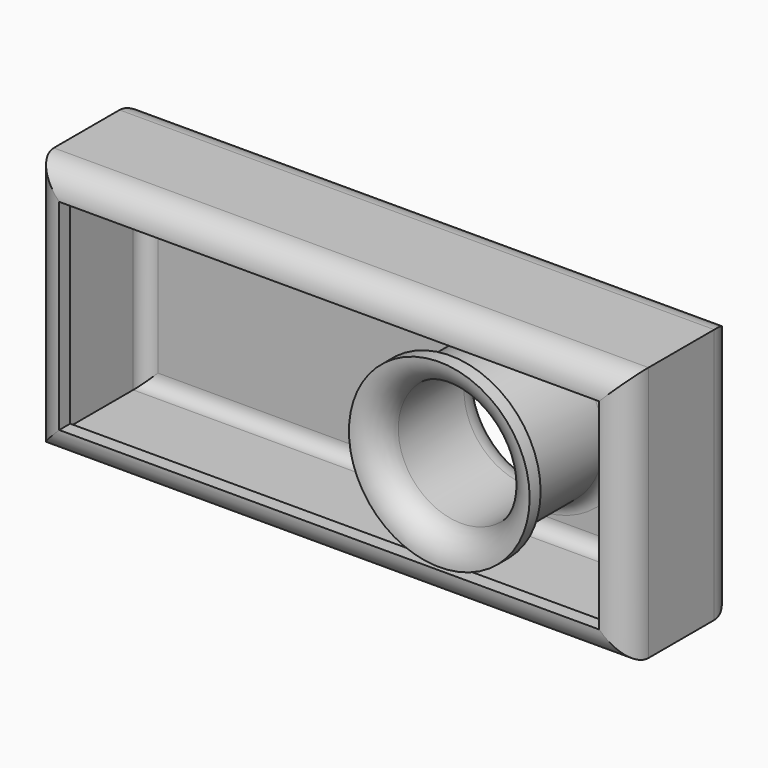
from build123d import *

# Parameters (mm, degrees)
F0_W     = 110.236
F0_H     = 47.3964
F1_DEPTH = 25.4
F2_R     = 11.6713
F3_DEPTH = 25.4
F4_R     = 5.08
F5_R     = 5.08
F6_T     = -2.54


# Not quite as in the source:
# - a shell that OpenCascade refuses in one call is made with other operations: the cavity is built on its own and cut out


with BuildPart() as f1:
    # F0 (on Front) → F1 (new body)
    with BuildSketch(Plane.XZ):
        with Locations((-0.954773277, -8.9795228673)):
            Rectangle(F0_W, F0_H)
    extrude(amount=F1_DEPTH)

    # F2 (on face) → F3 (cut, through all)
    with BuildSketch(Plane.XZ.offset(25.4)):
        with Locations((19.4582305849, -10.3191519156)):
            Circle(F2_R)
    extrude(amount=-F3_DEPTH, mode=Mode.SUBTRACT)

    # F4
    f4_edges = [f1.edges().sort_by_distance(p)[0] for p in [
        (7.786931, -25.4, -10.319152),
        (-0.954773, -25.4, 14.718677),
        (54.163227, -25.4, -8.979523),
        (-0.954773, -25.4, -32.677723),
        (-56.072773, -25.4, -8.979523),
        (7.786931, 0, -10.319152),
    ]]
    fillet(f4_edges, radius=F4_R)

    # F5
    f5_edges = [f1.edges().sort_by_distance(p)[0] for p in [
        (-0.954773, 0, 14.718677),
        (-56.072773, 0, -8.979523),
        (-0.954773, 0, -32.677723),
        (54.163227, 0, -8.979523),
    ]]
    fillet(f5_edges, radius=F5_R)

    # F6: a shell. OpenCascade refuses it in one call, so the cavity is built on its own and cut out:
    # the body offset inwards by the wall thickness, plus a prism from it out through each open face.
    f6_core = offset(f1.part, amount=F6_T, mode=Mode.PRIVATE)
    f6_exits = [f6_core.faces().sort_by_distance(p)[0] for p in [
        (-7.280112, -22.86, -8.564415),
    ]]
    add(f6_core, mode=Mode.SUBTRACT)
    extrude(f6_exits, amount=-F6_T, mode=Mode.SUBTRACT)


solid = f1.part
